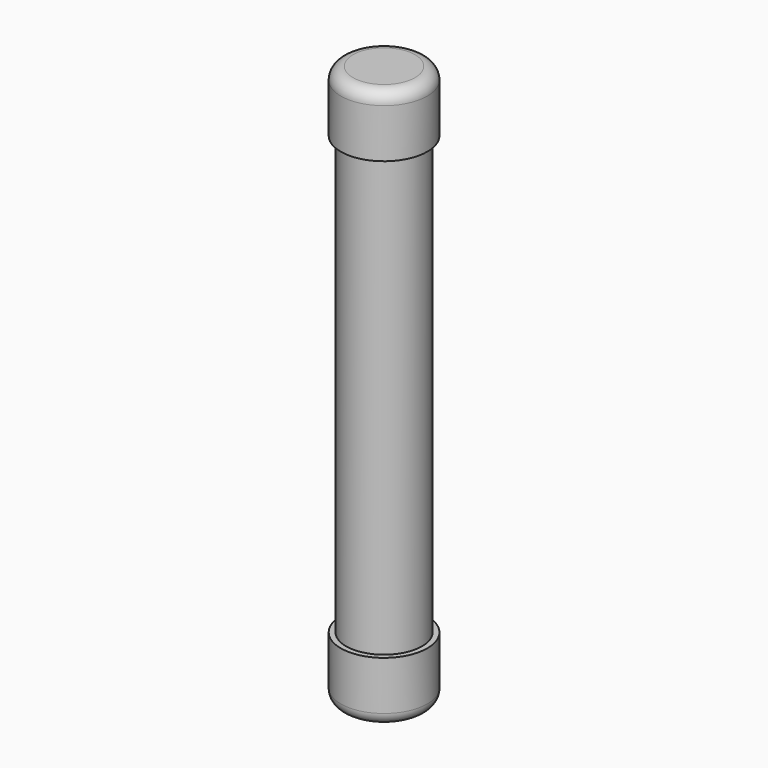
from build123d import *

# Parameters (mm, degrees)
F0_R          = 15.5
F1_DEPTH      = 114.3
F1_DEPTH_BACK = 114.3
F2_R          = 17.6785322686
F2_R_2        = 15.5
F3_DEPTH      = 25
F4_R          = 5


# Not quite as in the source:
# - a pattern or mirror of a feature is missing from the dataset's text; its kind, count and spacing are read off the source's solid


with BuildPart() as f1:
    # F0 (on Top) → F1 (new body, two sides)
    with BuildSketch(Plane.XY) as f1_sk:
        Circle(F0_R)
    extrude(amount=F1_DEPTH)
    extrude(f1_sk.sketch, amount=-F1_DEPTH_BACK)

    # F2 (on face) → F3 (join)
    with BuildSketch(Plane.XY.offset(114.3)):
        Circle(F2_R)
        Circle(F2_R_2, mode=Mode.SUBTRACT)
        Circle(F2_R_2)
    f3 = extrude(amount=-F3_DEPTH)

    # F3_copies: F3 across plane
    add(f3.mirror(Plane(origin=(0, 0, 0), x_dir=(-1, 0, 0), z_dir=(0, 0, -1))))

    # F4
    f4_edges = [f1.edges().sort_by_distance(p)[0] for p in [
        (-17.678532, 0, 114.3),
        (-17.678532, 0, -114.3),
    ]]
    fillet(f4_edges, radius=F4_R)


solid = f1.part
